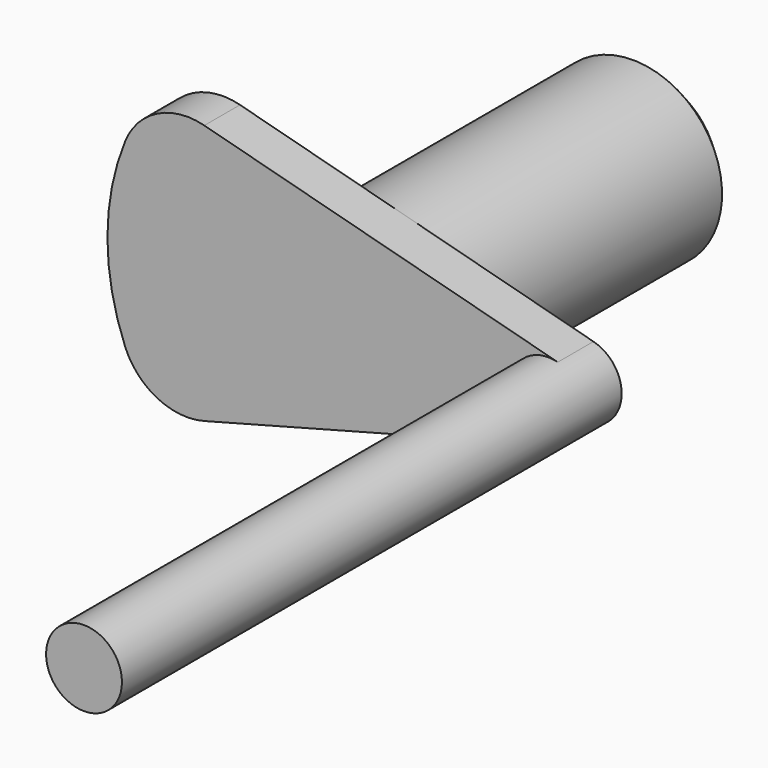
from build123d import *

# Parameters (mm, degrees)
F1_DEPTH = 2
F3_DEPTH = 26
F4_R     = 4
F5_DEPTH = 15
F6_SIZE  = 1


with BuildPart() as f1:
    # F0 (on Front) → F1 (new body)
    with BuildSketch(Plane.XZ):
        with BuildLine():
            ThreePointArc((9.4344444444, -1.6435504327), (10.3469512901, -1.0371702957), (10.7, 0))
            ThreePointArc((10.7, 0), (10.3469512901, 1.0371702957), (9.4344444444, 1.6435504327))
            Line((9.4344444444, 1.6435504327), (-6.407798527, 5.8311763854))
            ThreePointArc((-6.407798527, 5.8311763854), (-8.5124333236, 5.6159080306), (-9.9516775266, 4.0652938892))
            ThreePointArc((-9.9516775266, 4.0652938892), (-10.5485314952, 2.0714688736), (-10.75, 0))
            ThreePointArc((-10.75, 0), (-10.5485314952, -2.0714688736), (-9.9516775266, -4.0652938892))
            ThreePointArc((-9.9516775266, -4.0652938892), (-8.5124333236, -5.6159080306), (-6.407798527, -5.8311763854))
            Line((-6.407798527, -5.8311763854), (9.4344444444, -1.6435504327))
        make_face()
    extrude(amount=F1_DEPTH)

    # F2 (on face) → F3 (join)
    with BuildSketch(Plane.XZ.offset(2)):
        with BuildLine():
            ThreePointArc((9.4344444444, -1.6435504327), (10.3469512901, -1.0371702957), (10.7, 0))
            ThreePointArc((10.7, 0), (10.3469512901, 1.0371702957), (9.4344444444, 1.6435504327))
            ThreePointArc((9.4344444444, 1.6435504327), (7.3, 0), (9.4344444444, -1.6435504327))
        make_face()
    extrude(amount=F3_DEPTH)

    # F4 (on face) → F5 (join)
    with BuildSketch(Plane(origin=(0, 0, 0), x_dir=(-1, 0, 0), z_dir=(0, 1, 0))):
        Circle(F4_R)
    extrude(amount=F5_DEPTH)

    # F6
    f6_edges = [f1.edges().sort_by_distance(p)[0] for p in [
        (4, 15, 0),
    ]]
    chamfer(f6_edges, length=F6_SIZE)


solid = f1.part
